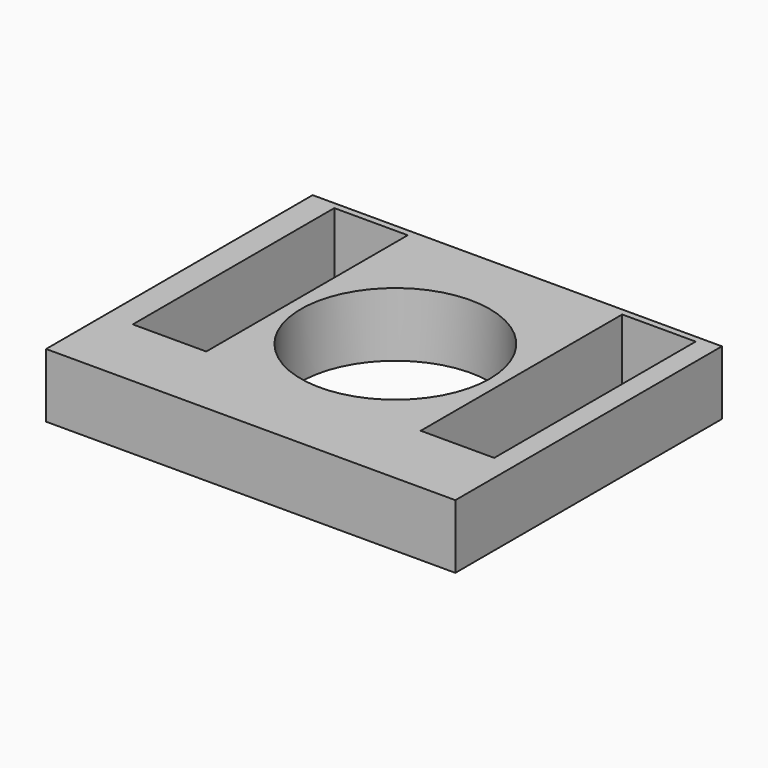
from build123d import *

# Parameters (mm, degrees)
F0_W     = 1981.2
F0_H     = 1612.9
F0_W_2   = 355.6
F0_H_2   = 1219.2
F0_R     = 457.2
F1_DEPTH = 101.6
F2_DEPTH = 208.28


# Not quite as in the source:
# - the program builds the solid bodies; features that only make, move or delete a surface that nothing else refers to are left out


with BuildPart() as f1:
    # F0 (on Top) → F1 (new body)
    with BuildSketch(Plane.XY):
        with Locations((-228.6, -50.8)):
            Rectangle(F0_W, F0_H)
        with Locations((-911.225, 114.3)):
            Rectangle(F0_W_2, F0_H_2, mode=Mode.SUBTRACT)
        with Locations((-214.3125, 0)):
            Circle(F0_R, mode=Mode.SUBTRACT)
        with Locations((482.6, 114.3)):
            Rectangle(F0_W_2, F0_H_2, mode=Mode.SUBTRACT)
    extrude(amount=F1_DEPTH)

    # F2 (add): a face of the model
    f2_faces = [f1.faces().sort_by_distance(p)[0] for p in [
        (736.4527890955, -50.8, 101.6),
    ]]
    extrude(f2_faces, amount=F2_DEPTH)


solid = f1.part
